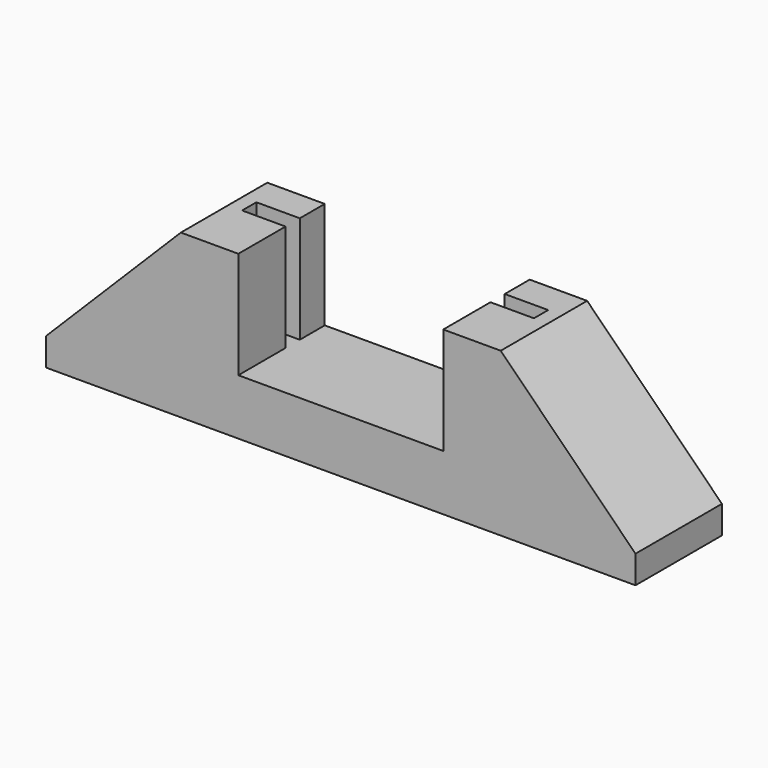
from build123d import *

# Parameters (mm, degrees)
F0_W      = 4.572
F0_H      = 2.032
F1_DEPTH  = 1.6
F3_DEPTH  = 12.192
F4_DEPTH  = 3.175
F5_DEPTH  = 0.508
F6_DEPTH  = 0.508
F7_DEPTH  = 0.508
F8_DEPTH  = 0.508
F9_DEPTH  = 0.127
F11_DEPTH = 1.5875
F13_DEPTH = 12.319
F14_DEPTH = 3.175


# Not quite as in the source:
# - a feature of the source that left no trace in its solid (it failed there, or was rolled back) is left out
# - a pattern or mirror of a feature is missing from the dataset's text; its kind, count and spacing are read off the source's solid


with BuildPart() as f1:
    # F0 (on Top) → F1 (new body)
    with BuildSketch(Plane.XY):
        Polygon((0, -2.032), (0, 0), (4.572, 0), (4.572, 3.556), (-1.6, 3.556), (-1.6, -1.016), (-1.6, -5.588), (4.572, -5.588), (4.572, -2.032), align=None)
        Polygon((33.858, 3.556), (27.686, 3.556), (27.686, 0), (32.258, 0), (32.258, -2.032), (27.686, -2.032), (27.686, -5.588), (33.858, -5.588), (33.858, -1.016), align=None)
        Polygon((4.572, 3.556), (4.572, 0), (4.572, -2.032), (4.572, -5.588), (27.686, -5.588), (27.686, -2.032), (27.686, 0), (27.686, 3.556), align=None)
        with Locations((2.286, -1.016)):
            Rectangle(F0_W, F0_H)
        with Locations((29.972, -1.016)):
            Rectangle(F0_W, F0_H)
    extrude(amount=F1_DEPTH)

    # F2 (on face) → F3 (join)
    with BuildSketch(Plane.XY.offset(1.6)):
        Polygon((0, -2.032), (0, 0), (4.572, 0), (4.572, 3.556), (-1.6, 3.556), (-1.6, -1.016), (-1.6, -5.588), (4.572, -5.588), (4.572, -2.032), align=None)
        Polygon((33.858, 3.556), (27.686, 3.556), (27.686, 0), (32.258, 0), (32.258, -2.032), (27.686, -2.032), (27.686, -5.588), (33.858, -5.588), (33.858, -1.016), align=None)
    extrude(amount=F3_DEPTH)

    # F4 (add): a face of the model
    f4_faces = [f1.faces().sort_by_distance(p)[0] for p in [
        (-1.2195411943, -5.588, 6.896),
    ]]
    extrude(f4_faces, amount=F4_DEPTH)

    # F5 (add): a face of the model
    f5_faces = [f1.faces().sort_by_distance(p)[0] for p in [
        (-1.6, -2.6035, 6.896),
    ]]
    extrude(f5_faces, amount=F5_DEPTH)

    # F6 (cut): a face of the model
    f6_faces = [f1.faces().sort_by_distance(p)[0] for p in [
        (0, -1.016, 7.696),
    ]]
    extrude(f6_faces, amount=-F6_DEPTH, mode=Mode.SUBTRACT)

    # F7 (add): a face of the model
    f7_faces = [f1.faces().sort_by_distance(p)[0] for p in [
        (33.858, -2.6035, 6.896),
    ]]
    extrude(f7_faces, amount=F7_DEPTH)

    # F8 (cut): a face of the model
    f8_faces = [f1.faces().sort_by_distance(p)[0] for p in [
        (32.258, -1.016, 7.696),
    ]]
    extrude(f8_faces, amount=-F8_DEPTH, mode=Mode.SUBTRACT)

    # F9 (cut): faces of the model
    f9_faces = [f1.faces().sort_by_distance(p)[0] for p in [
        (4.572, -5.3975, 7.696),
        (4.572, 1.778, 7.696),
    ]]
    f9 = extrude(f9_faces, amount=-F9_DEPTH, mode=Mode.SUBTRACT)

    # F9_copies: F9 across plane
    add(f9.mirror(Plane(origin=(16.129, 0, 0), x_dir=(0, 0, 1), z_dir=(1, 0, 0))), mode=Mode.SUBTRACT)

    # F11 (add): a face of the model
    f11_faces = [f1.faces().sort_by_distance(p)[0] for p in [
        (16.129, -2.6035, 0),
    ]]
    extrude(f11_faces, amount=F11_DEPTH)

    # F12 (on face) → F13 (join, through all)
    with BuildSketch(Plane.XZ.offset(8.763)):
        Polygon((-2.108, -1.5875), (-2.108, 13.792), (-17.475, -1.5875), align=None)
        Polygon((49.733, -1.5875), (34.366, 13.792), (34.366, -1.5875), align=None)
    extrude(amount=-F13_DEPTH)

    # F14 (add): a face of the model
    f14_faces = [f1.faces().sort_by_distance(p)[0] for p in [
        (16.129, -2.6035, -1.5875),
    ]]
    extrude(f14_faces, amount=F14_DEPTH)


solid = f1.part
